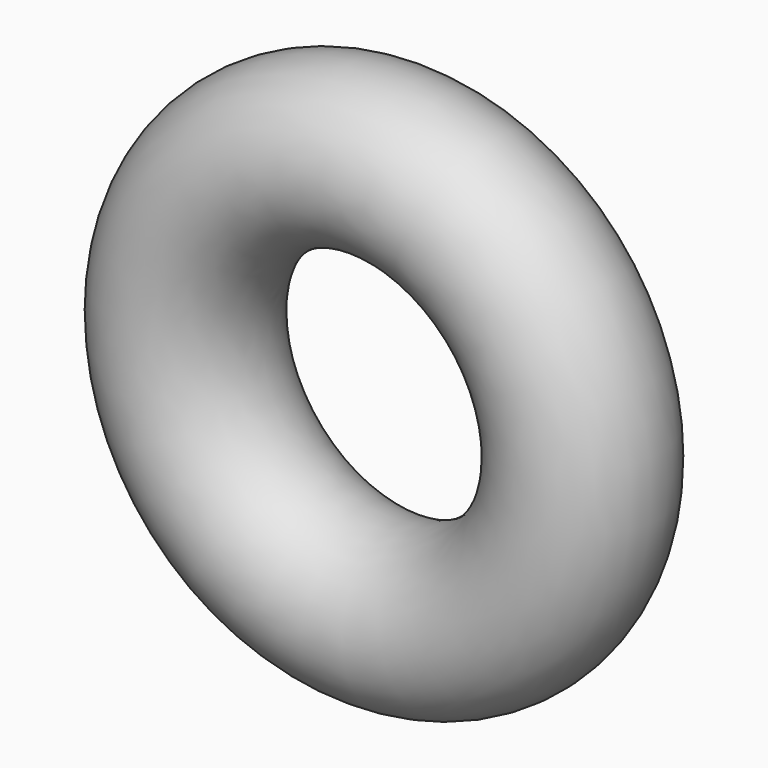
from build123d import *

# Parameters (mm, degrees)
F3_R = 12.0761533709


# Not quite as in the source:
# - the program builds the solid bodies; features that only make, move or delete a surface that nothing else refers to are left out


with BuildPart() as f4:
    # F3 (on Right) → F4 (revolve)
    with BuildSketch(Plane.YZ):
        with Locations((-38.636893034, 6.7262914963)):
            Circle(F3_R)
    revolve(axis=Axis((0, -38.6390378699, 37.1608063579), (0, 1, 0)))


solid = f4.part
